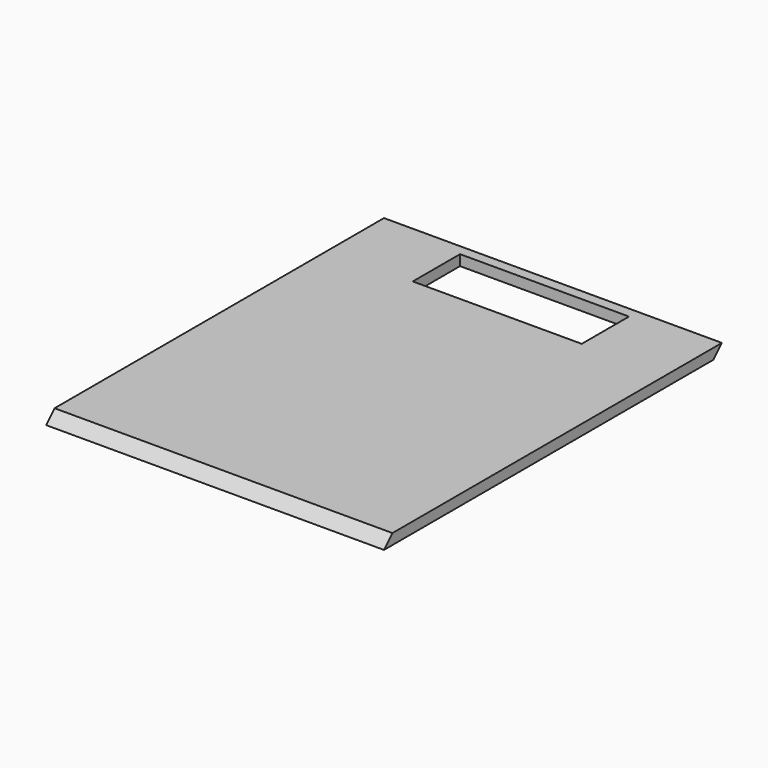
from build123d import *

# Parameters (mm, degrees)
F0_W     = 101.6
F0_H     = 127
F1_DEPTH = 3.175
F2_SIZE  = 3.17499
F3_SIZE  = 3.17499
F4_W     = 31.75
F4_H     = 17.7633663237
F4_W_2   = 19.05
F5_DEPTH = 3.175


# Not quite as in the source:
# - a fillet or chamfer is up to 0.001 mm smaller than in the source, because OpenCascade refuses the exact size
# - a length typed as a fraction of an inch, garbled in the dataset ("3 / 203.2 mm" for 3/8 in), is restored


with BuildPart() as f1:
    # F0 (on Top) → F1 (new body)
    with BuildSketch(Plane.XY):
        with Locations((5.2556597352, 10.8384059966)):
            Rectangle(F0_W, F0_H)
    extrude(amount=F1_DEPTH)

    # F2 (size 3.175 in the source; OpenCascade refuses exactly that, so slightly less here)
    f2_edges = [f1.edges().sort_by_distance(p)[0] for p in [
        (5.25566, 74.338406, 0),
    ]]
    chamfer(f2_edges, length=F2_SIZE)

    # F3 (size 3.175 in the source; OpenCascade refuses exactly that, so slightly less here)
    f3_edges = [f1.edges().sort_by_distance(p)[0] for p in [
        (5.25566, -52.661594, 3.175),
    ]]
    chamfer(f3_edges, length=F3_SIZE)

    # F4 (on face) → F5 (cut)
    with BuildSketch(Plane(origin=(0, 0, 0), x_dir=(1, 0, 0), z_dir=(0, 0, -1))):
        with Locations((-4.2693402648, -62.2817228347)):
            Rectangle(F4_W, F4_H)
        with Locations((21.1306597352, -62.2817228347)):
            Rectangle(F4_W_2, F4_H)
    extrude(amount=-F5_DEPTH, mode=Mode.SUBTRACT)


solid = f1.part
